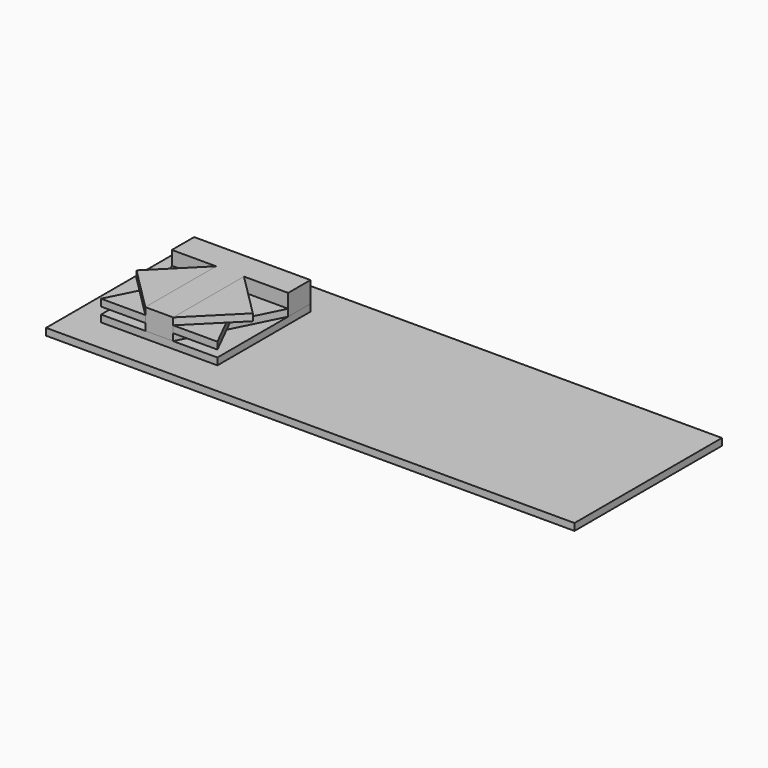
from build123d import *

# Parameters (mm, degrees)
F0_W      = 192.7787214518
F0_H      = 67.2237873077
F1_DEPTH  = 2.54
F2_W      = 42.4414947629
F2_H      = 42.4414947629
F3_DEPTH  = 2.54
F5_DEPTH  = 7.62
F7_DEPTH  = 2.54
F9_DEPTH  = 2.54
F11_DEPTH = 2.54


# Not quite as in the source:
# - a feature names something its author has since deleted; it is built from what else it names


with BuildPart() as f1:
    # F0 (on Top) → F1 (new body)
    with BuildSketch(Plane.XY):
        Rectangle(F0_W, F0_H)
    extrude(amount=F1_DEPTH)


with BuildPart() as f3:
    # F2 (on face) → F3 (new body)
    with BuildSketch(Plane.XY.offset(2.54)):
        with Locations((-65.0134757161, 0)):
            Rectangle(F2_W, F2_H)
    extrude(amount=F3_DEPTH)

    # F6 (on face) → F7 (join)
    with BuildSketch(Plane.XY.offset(5.08)):
        Polygon((-70.0934757161, 11.0607473814), (-86.2342230976, 11.0607473814), (-70.0934757161, -21.2207473814), align=None)
        Polygon((-59.9334757161, 11.0607473814), (-59.9334757161, -21.2207473814), (-43.7927283347, 11.0607473814), align=None)
    extrude(amount=F7_DEPTH)

    # F8 (on face) → F9 (join)
    with BuildSketch(Plane.XY.offset(7.62)):
        Polygon((-86.2342230976, -21.2207473814), (-70.0934757161, -21.2207473814), (-70.0934757161, 11.0607473814), align=None)
        Polygon((-59.9334757161, 11.0607473814), (-59.9334757161, -21.2207473814), (-43.7927283347, -21.2207473814), align=None)
    extrude(amount=F9_DEPTH)

    # F10 (on face) → F11 (join)
    with BuildSketch(Plane.XY.offset(10.16)):
        Polygon((-70.0934757161, -21.2207473814), (-70.0934757161, 11.0607473814), (-86.2342230976, -5.08), align=None)
        Polygon((-59.9334757161, 11.0607473814), (-59.9334757161, -21.2207473814), (-43.7927283347, -5.08), align=None)
    extrude(amount=F11_DEPTH)


with BuildPart() as f5:
    # F4 (on face) → F5 (new body)
    with BuildSketch(Plane.XY.offset(5.08)):
        Polygon((-43.7927283347, 21.2207473814), (-86.2342230976, 21.2207473814), (-86.2342230976, 11.0607473814), (-70.0934757161, 11.0607473814), (-70.0934757161, -21.2207473814), (-59.9334757161, -21.2207473814), (-59.9334757161, 11.0607473814), (-43.7927283347, 11.0607473814), align=None)
    extrude(amount=F5_DEPTH)


solid = Compound([f1.part, f3.part, f5.part])
